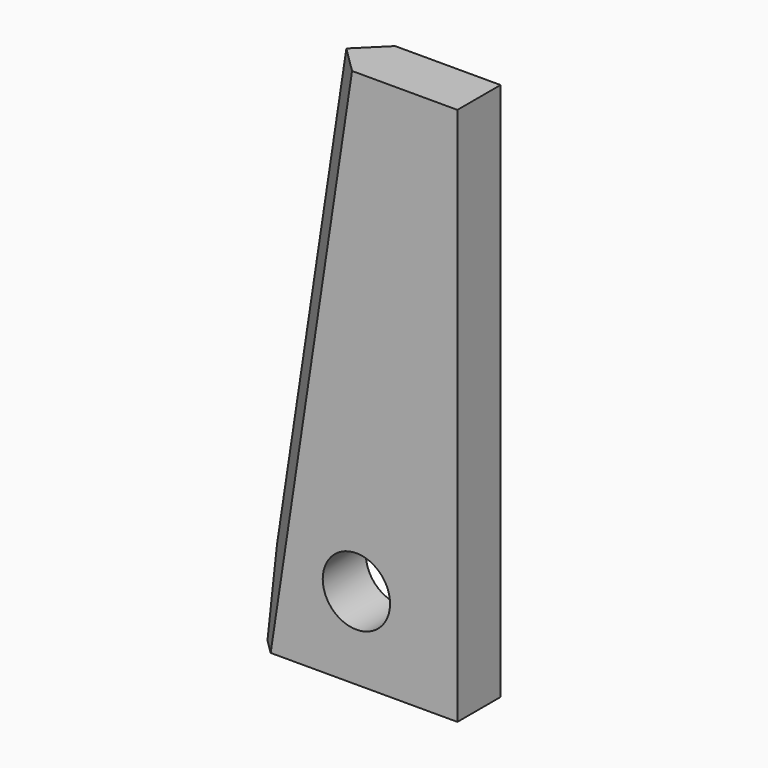
from build123d import *

# Parameters (mm, degrees)
F0_W     = 19.05
F0_H     = 50.8
F1_DEPTH = 5.08
F3_D     = 6.35
F5_DEPTH = 25.4
F6_SIZE  = 2.53999


# Not quite as in the source:
# - a fillet or chamfer is up to 0.001 mm smaller than in the source, because OpenCascade refuses the exact size


with BuildPart() as f1:
    # F0 (on Front) → F1 (new body)
    with BuildSketch(Plane.XZ):
        with Locations((-9.525, 25.4)):
            Rectangle(F0_W, F0_H)
    extrude(amount=F1_DEPTH)

    # F3 (through all)
    with Locations(Plane.XZ.offset(5.08)):
        with Locations((-9.525, 7.7354544774)):
            Hole(F3_D / 2)

    # F4 (on face) → F5 (cut)
    with BuildSketch(Plane.XZ.offset(5.08)):
        Polygon((-19.05, 7.4566449039), (-12.5023688375, 50.8), (-19.05, 50.8), align=None)
    extrude(amount=-F5_DEPTH, mode=Mode.SUBTRACT)

    # F6 (size 2.54 in the source; OpenCascade refuses exactly that, so slightly less here)
    f6_edges = [f1.edges().sort_by_distance(p)[0] for p in [
        (-15.776184, -5.08, 29.128322),
        (-15.776184, 0, 29.128322),
    ]]
    chamfer(f6_edges, length=F6_SIZE)


solid = f1.part
